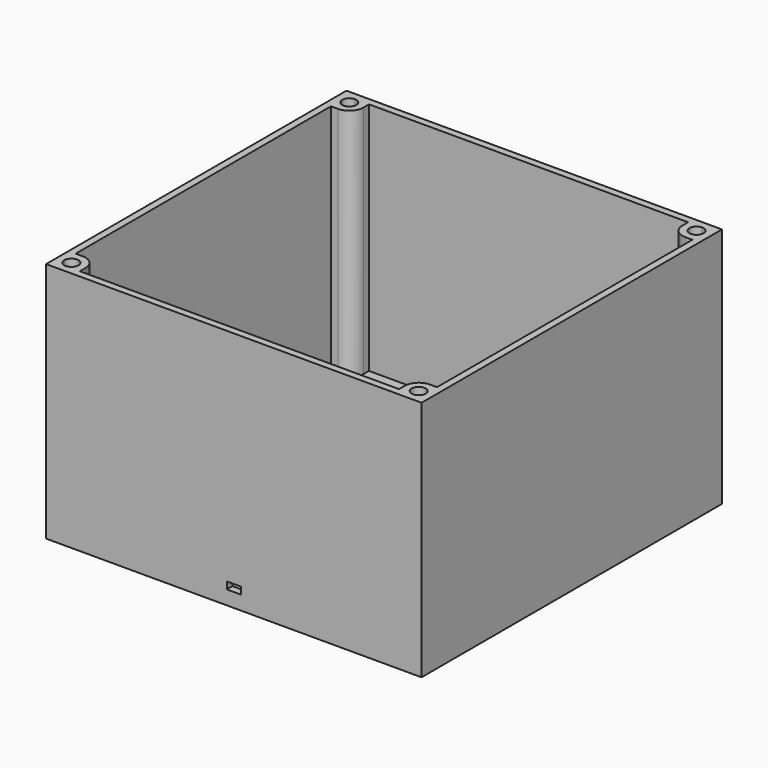
from build123d import *

# Parameters (mm, degrees)
F0_W     = 80
F0_H     = 80
F1_DEPTH = 51.5
F2_T     = -1.5
F4_DEPTH = 50
F5_W     = 3
F5_H     = 1.5
F6_DEPTH = 1.5


with BuildPart() as f1:
    # F0 (on Top) → F1 (new body)
    with BuildSketch(Plane.XY):
        Rectangle(F0_W, F0_H)
    extrude(amount=F1_DEPTH)

    # F2
    f2_openings = [f1.faces().sort_by_distance(p)[0] for p in [
        (0, 0, 51.5),
    ]]
    offset(amount=F2_T, openings=f2_openings)

    # F3 (on face) → F4 (join, through all)
    with BuildSketch(Plane.XY.offset(51.5)):
        with BuildLine():
            ThreePointArc((-36.9999999833, 38.5), (-35.9393398223, 38.0606601659), (-35.5, 37))
            ThreePointArc((-35.5, 37), (-37, 35.5), (-38.5, 37))
            Line((-38.5, 37), (-38.5, 34))
            Line((-38.5, 34), (-37, 34))
            ThreePointArc((-37, 34), (-34.8786796564, 34.8786796564), (-34, 37))
            Line((-34, 37), (-34, 38.5))
            Line((-34, 38.5), (-36.9999999833, 38.5))
        make_face()
        with BuildLine():
            ThreePointArc((-38.5, 37), (-38.0606601659, 38.0606601777), (-36.9999999833, 38.5))
            Line((-36.9999999833, 38.5), (-38.5, 38.5))
            Line((-38.5, 38.5), (-38.5, 37))
        make_face()
        with BuildLine():
            Line((-37, -34), (-38.5, -34))
            Line((-38.5, -34), (-38.5, -37))
            ThreePointArc((-38.5, -37), (-37, -35.5), (-35.5, -37))
            ThreePointArc((-35.5, -37), (-35.9393398378, -38.0606601813), (-37.0000000271, -38.5))
            Line((-37.0000000271, -38.5), (-34, -38.5))
            Line((-34, -38.5), (-34, -37))
            ThreePointArc((-34, -37), (-34.8786796564, -34.8786796564), (-37, -34))
        make_face()
        with BuildLine():
            ThreePointArc((-37.0000000271, -38.5), (-38.0606601813, -38.0606601622), (-38.5, -37))
            Line((-38.5, -37), (-38.5, -38.5))
            Line((-38.5, -38.5), (-37.0000000271, -38.5))
        make_face()
        with BuildLine():
            Line((38.5, -37), (38.5, -34))
            Line((38.5, -34), (37, -34))
            ThreePointArc((37, -34), (34.8786796564, -34.8786796564), (34, -37))
            Line((34, -37), (34, -38.5))
            Line((34, -38.5), (37, -38.5))
            ThreePointArc((37, -38.5), (35.9393398282, -35.9393398282), (38.5, -37))
        make_face()
        with BuildLine():
            Line((38.5, -38.5), (38.5, -37))
            ThreePointArc((38.5, -37), (38.0606601718, -38.0606601718), (37, -38.5))
            Line((37, -38.5), (38.5, -38.5))
        make_face()
        with BuildLine():
            Line((37.0000000167, 38.5), (34, 38.5))
            Line((34, 38.5), (34, 37))
            ThreePointArc((34, 37), (34.8786796564, 34.8786796564), (37, 34))
            Line((37, 34), (38.5, 34))
            Line((38.5, 34), (38.5, 37))
            ThreePointArc((38.5, 37), (35.9393398223, 35.9393398341), (37.0000000167, 38.5))
        make_face()
        with BuildLine():
            Line((38.5, 38.5), (37.0000000167, 38.5))
            ThreePointArc((37.0000000167, 38.5), (38.0606601777, 38.0606601659), (38.5, 37))
            Line((38.5, 37), (38.5, 38.5))
        make_face()
    extrude(amount=-F4_DEPTH)

    # F5 (on face) → F6 (cut, through all)
    with BuildSketch(Plane.XZ.offset(40)):
        with Locations((0, 3.75)):
            Rectangle(F5_W, F5_H)
    extrude(amount=-F6_DEPTH, mode=Mode.SUBTRACT)


solid = f1.part
